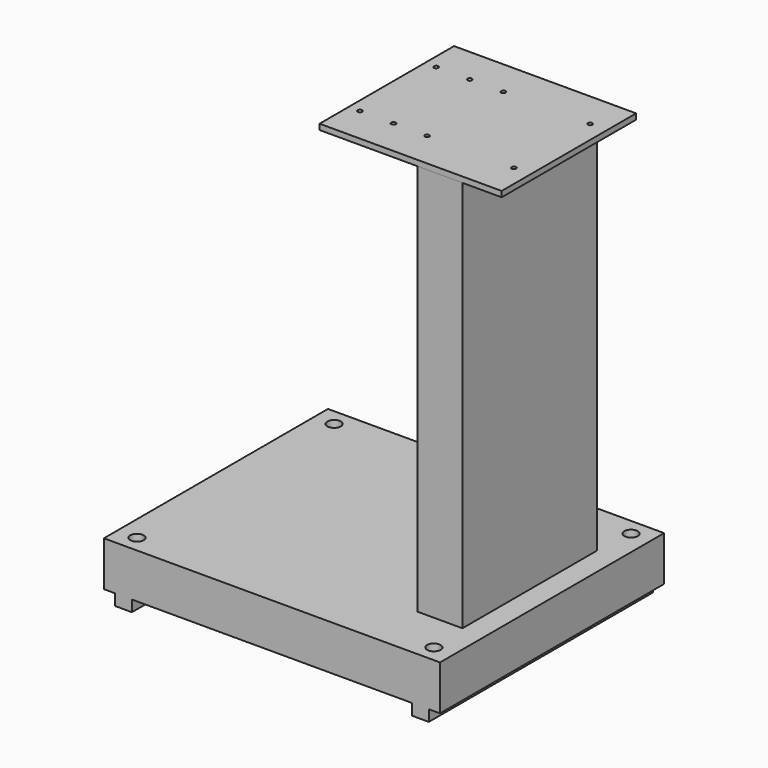
from build123d import *

# Parameters (mm, degrees)
F1_DEPTH  = 500
F4_R      = 12
F3_R      = 12
F5_DEPTH  = 100.001
F2_W      = 80
F2_H      = 300
F6_DEPTH  = 700
F7_W      = 80
F7_H      = 300
F7_W_2    = 175
F7_W_3    = 70
F8_DEPTH  = 10
F9_R      = 4
F10_DEPTH = 10


with BuildPart() as f1:
    # F0 (on Front) → F1 (new body)
    with BuildSketch(Plane.XZ):
        Polygon((336.7550126589, 80), (-263.2449873411, 80), (-263.2449873411, 0), (-243.2449873411, 0), (-243.2449873411, -20), (-213.2449873411, -20), (-213.2449873411, 0), (286.7550126589, 0), (286.7550126589, -20), (316.7550126589, -20), (316.7550126589, 0), (336.7550126589, 0), align=None)
    extrude(amount=F1_DEPTH)

    # F4 (on face) + F3 (on face) → F5 (cut, through all)
    with BuildSketch(Plane(origin=(0, 0, -20), x_dir=(1, 0, 0), z_dir=(0, 0, -1))):
        with Locations((301.7550126589, 470)):
            Circle(F4_R)
        with Locations((301.7550126589, 30)):
            Circle(F4_R)
    with BuildSketch(Plane(origin=(0, 0, -20), x_dir=(1, 0, 0), z_dir=(0, 0, -1))):
        with Locations((-228.2449873411, 30)):
            Circle(F3_R)
        with Locations((-228.2449873411, 470)):
            Circle(F3_R)
    extrude(amount=-F5_DEPTH, mode=Mode.SUBTRACT)


with BuildPart() as f6:
    # F2 (on face) → F6 (new body)
    with BuildSketch(Plane.XY.offset(80)):
        with Locations((256.7550126589, -250)):
            Rectangle(F2_W, F2_H)
    extrude(amount=F6_DEPTH)


with BuildPart() as f8:
    # F7 (on face) → F8 (new body)
    with BuildSketch(Plane.XY.offset(780)):
        with Locations((256.7550126589, -250)):
            Rectangle(F7_W, F7_H)
        with Locations((129.2550126589, -250)):
            Rectangle(F7_W_2, F7_H)
        with Locations((331.7550126589, -250)):
            Rectangle(F7_W_3, F7_H)
    extrude(amount=F8_DEPTH)

    # F9 (on face) → F10 (cut)
    with BuildSketch(Plane.XY.offset(790)):
        with Locations((121.7550126589, -335)):
            Circle(F9_R)
        with Locations((61.7550126589, -335)):
            Circle(F9_R)
        with Locations((181.7550126589, -335)):
            Circle(F9_R)
        with Locations((336.7550126589, -335)):
            Circle(F9_R)
        with Locations((336.7550126589, -165)):
            Circle(F9_R)
        with Locations((181.7550126589, -165)):
            Circle(F9_R)
        with Locations((121.7550126589, -165)):
            Circle(F9_R)
        with Locations((61.7550126589, -165)):
            Circle(F9_R)
    extrude(amount=-F10_DEPTH, mode=Mode.SUBTRACT)


solid = Compound([f1.part, f6.part, f8.part])
